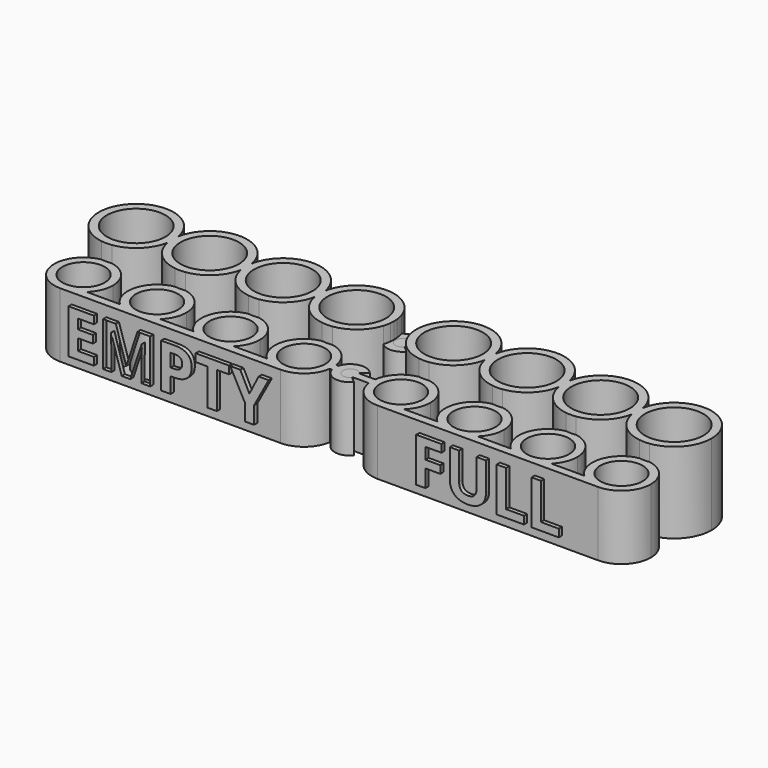
from build123d import *

# Parameters (mm, degrees)
F0_R         = 7.25
F1_DEPTH     = 20
F0_R_2       = 5.25
F2_DEPTH     = 16
F3_DEPTH     = 1.6
F4_TEXT_SIZE = 15.2777777778
F5_DEPTH     = 1
F6_DEPTH     = 20
F7_DEPTH     = 16
F8_TEXT_SIZE = 15.2777777778
F9_DEPTH     = 1
F10_DEPTH    = 1.6


# Not quite as in the source:
# - a feature names something its author has since deleted; it is built from what else it names
# - Text() gives the source's letters only with a copy of the font that has no kerning and outlines rounded to 1/6400 em; it was checked with that copy


with BuildPart() as f1:
    # F0 (on Top) → F1 (new body)
    with BuildSketch(Plane.XY):
        with BuildLine():
            ThreePointArc((-15.1805921053, -2.7893627205), (-16.4, 0), (-15.1805921053, 2.7893627205))
            ThreePointArc((-15.1805921053, 2.7893627205), (-24.5823020266, 9.231653392), (-33.1, 1.6590660023))
            ThreePointArc((-33.1, 1.6590660023), (-32.9875763232, 0.8329165624), (-32.95, 0))
            ThreePointArc((-32.95, 0), (-32.9875763232, -0.8329165624), (-33.1, -1.6590660023))
            ThreePointArc((-33.1, -1.6590660023), (-30.4002858895, -6.678236334), (-25.2709482961, -9.1622699387))
            ThreePointArc((-25.2709482961, -9.1622699387), (-24, -9.05), (-22.7290517039, -9.1622699387))
            ThreePointArc((-22.7290517039, -9.1622699387), (-18.0328140118, -7.067898654), (-15.1805921053, -2.7893627205))
        make_face()
        with Locations((-24, 0)):
            Circle(F0_R, mode=Mode.SUBTRACT)
        with BuildLine():
            ThreePointArc((-14.8042129211, 1), (-14.9480793629, 1.9040044063), (-15.1805921053, 2.7893627205))
            ThreePointArc((-15.1805921053, 2.7893627205), (-16.4, 0), (-15.1805921053, -2.7893627205))
            ThreePointArc((-15.1805921053, -2.7893627205), (-14.9480793629, -1.9040044063), (-14.8042129211, -1))
            ThreePointArc((-14.8042129211, -1), (-14.763563174, -0.5007342211), (-14.75, 0))
            ThreePointArc((-14.75, 0), (-14.763563174, 0.5007342211), (-14.8042129211, 1))
        make_face()
        with BuildLine():
            ThreePointArc((-32.95, 0), (-32.9875763232, 0.8329165624), (-33.1, 1.6590660023))
            ThreePointArc((-33.1, 1.6590660023), (-33.25, 0), (-33.1, -1.6590660023))
            ThreePointArc((-33.1, -1.6590660023), (-32.9875763232, -0.8329165624), (-32.95, 0))
        make_face()
        with BuildLine():
            ThreePointArc((-33.1, -1.6590660023), (-33.25, 0), (-33.1, 1.6590660023))
            ThreePointArc((-33.1, 1.6590660023), (-42.2, 9.25), (-51.3, 1.6590660023))
            ThreePointArc((-51.3, 1.6590660023), (-51.1875763232, 0.8329165624), (-51.15, 0))
            ThreePointArc((-51.15, 0), (-51.1875763232, -0.8329165624), (-51.3, -1.6590660023))
            ThreePointArc((-51.3, -1.6590660023), (-48.6002858895, -6.678236334), (-43.4709482961, -9.1622699387))
            ThreePointArc((-43.4709482961, -9.1622699387), (-42.2, -9.05), (-40.9290517039, -9.1622699387))
            ThreePointArc((-40.9290517039, -9.1622699387), (-35.7997141105, -6.678236334), (-33.1, -1.6590660023))
        make_face()
        with Locations((-42.2, 0)):
            Circle(F0_R, mode=Mode.SUBTRACT)
        with BuildLine():
            ThreePointArc((-25.2709482961, -9.1622699387), (-24, -9.25), (-22.7290517039, -9.1622699387))
            ThreePointArc((-22.7290517039, -9.1622699387), (-24, -9.05), (-25.2709482961, -9.1622699387))
        make_face()
        with BuildLine():
            ThreePointArc((-51.15, 0), (-51.1875763232, 0.8329165624), (-51.3, 1.6590660023))
            ThreePointArc((-51.3, 1.6590660023), (-51.45, 0), (-51.3, -1.6590660023))
            ThreePointArc((-51.3, -1.6590660023), (-51.1875763232, -0.8329165624), (-51.15, 0))
        make_face()
        with BuildLine():
            ThreePointArc((-51.3, -1.6590660023), (-51.45, 0), (-51.3, 1.6590660023))
            ThreePointArc((-51.3, 1.6590660023), (-60.4, 9.25), (-69.5, 1.6590660023))
            ThreePointArc((-69.5, 1.6590660023), (-69.3875763232, 0.8329165624), (-69.35, 0))
            ThreePointArc((-69.35, 0), (-69.3875763232, -0.8329165624), (-69.5, -1.6590660023))
            ThreePointArc((-69.5, -1.6590660023), (-66.8002858895, -6.678236334), (-61.6709482961, -9.1622699387))
            ThreePointArc((-61.6709482961, -9.1622699387), (-60.4, -9.05), (-59.1290517039, -9.1622699387))
            ThreePointArc((-59.1290517039, -9.1622699387), (-53.9997141105, -6.678236334), (-51.3, -1.6590660023))
        make_face()
        with Locations((-60.4, 0)):
            Circle(F0_R, mode=Mode.SUBTRACT)
        with BuildLine():
            ThreePointArc((-43.4709482961, -9.1622699387), (-42.2, -9.25), (-40.9290517039, -9.1622699387))
            ThreePointArc((-40.9290517039, -9.1622699387), (-42.2, -9.05), (-43.4709482961, -9.1622699387))
        make_face()
        with BuildLine():
            ThreePointArc((-69.35, 0), (-69.3875763232, 0.8329165624), (-69.5, 1.6590660023))
            ThreePointArc((-69.5, 1.6590660023), (-69.65, 0), (-69.5, -1.6590660023))
            ThreePointArc((-69.5, -1.6590660023), (-69.3875763232, -0.8329165624), (-69.35, 0))
        make_face()
        with BuildLine():
            ThreePointArc((-69.5, -1.6590660023), (-69.65, 0), (-69.5, 1.6590660023))
            ThreePointArc((-69.5, 1.6590660023), (-85.278236334, 6.4002858895), (-79.8709482961, -9.1622699387))
            ThreePointArc((-79.8709482961, -9.1622699387), (-78.6, -9.05), (-77.3290517039, -9.1622699387))
            ThreePointArc((-77.3290517039, -9.1622699387), (-72.1997141105, -6.678236334), (-69.5, -1.6590660023))
        make_face()
        with Locations((-78.6, 0)):
            Circle(F0_R, mode=Mode.SUBTRACT)
        with BuildLine():
            ThreePointArc((-61.6709482961, -9.1622699387), (-60.4, -9.25), (-59.1290517039, -9.1622699387))
            ThreePointArc((-59.1290517039, -9.1622699387), (-60.4, -9.05), (-61.6709482961, -9.1622699387))
        make_face()
        with BuildLine():
            ThreePointArc((-77.3290517039, -9.1622699387), (-78.6, -9.05), (-79.8709482961, -9.1622699387))
            ThreePointArc((-79.8709482961, -9.1622699387), (-78.6, -9.25), (-77.3290517039, -9.1622699387))
        make_face()
    extrude(amount=F1_DEPTH)

    # F0 (on Top) → F2 (join)
    with BuildSketch(Plane.XY):
        with BuildLine():
            Line((-16.266060556, -15.3), (-16.8192966918, -15.3))
            ThreePointArc((-16.8192966918, -15.3), (-16.767344921, -15.7988009299), (-16.75, -16.3))
            ThreePointArc((-16.75, -16.3), (-16.767344921, -16.8011990701), (-16.8192966918, -17.3))
            Line((-16.8192966918, -17.3), (-16.266060556, -17.3))
            ThreePointArc((-16.266060556, -17.3), (-16.4, -16.3), (-16.266060556, -15.3))
        make_face()
        with BuildLine():
            Line((-14.0966629547, -15.3), (-16.266060556, -15.3))
            ThreePointArc((-16.266060556, -15.3), (-16.4, -16.3), (-16.266060556, -17.3))
            Line((-16.266060556, -17.3), (-14.0966629547, -17.3))
            ThreePointArc((-14.0966629547, -17.3), (-14.4, -16.3), (-14.0966629547, -15.3))
        make_face()
        with BuildLine():
            ThreePointArc((-77.3290517039, -9.1622699387), (-78.6, -9.25), (-79.8709482961, -9.1622699387))
            ThreePointArc((-79.8709482961, -9.1622699387), (-85.8218779741, -16.9379486873), (-78.6, -23.55))
            ThreePointArc((-78.6, -23.55), (-75.9074175964, -23.0314560089), (-73.6, -21.55))
            ThreePointArc((-73.6, -21.55), (-71.9361985324, -19.1559149147), (-71.35, -16.3))
            ThreePointArc((-71.35, -16.3), (-73.0422632688, -11.6444589545), (-77.3290517039, -9.1622699387))
        make_face()
        with Locations((-78.6, -16.3)):
            Circle(F0_R_2, mode=Mode.SUBTRACT)
        with BuildLine():
            ThreePointArc((-73.6, -21.55), (-75.9074175964, -23.0314560089), (-78.6, -23.55))
            Line((-78.6, -23.55), (-60.4, -23.55))
            ThreePointArc((-60.4, -23.55), (-63.0925824036, -23.0314560089), (-65.4, -21.55))
            Line((-65.4, -21.55), (-73.6, -21.55))
        make_face()
        with BuildLine():
            ThreePointArc((-53.15, -16.3), (-54.8422632688, -11.6444589545), (-59.1290517039, -9.1622699387))
            ThreePointArc((-59.1290517039, -9.1622699387), (-60.4, -9.25), (-61.6709482961, -9.1622699387))
            ThreePointArc((-61.6709482961, -9.1622699387), (-67.3422735578, -14.2101823408), (-65.4, -21.55))
            ThreePointArc((-65.4, -21.55), (-63.0925824036, -23.0314560089), (-60.4, -23.55))
            ThreePointArc((-60.4, -23.55), (-57.7074175964, -23.0314560089), (-55.4, -21.55))
            ThreePointArc((-55.4, -21.55), (-53.7361985324, -19.1559149147), (-53.15, -16.3))
        make_face()
        with Locations((-60.4, -16.3)):
            Circle(F0_R_2, mode=Mode.SUBTRACT)
        with BuildLine():
            ThreePointArc((-42.2, -23.55), (-44.8925824036, -23.0314560089), (-47.2, -21.55))
            Line((-47.2, -21.55), (-55.4, -21.55))
            ThreePointArc((-55.4, -21.55), (-57.7074175964, -23.0314560089), (-60.4, -23.55))
            Line((-60.4, -23.55), (-42.2, -23.55))
        make_face()
        with BuildLine():
            ThreePointArc((-34.95, -16.3), (-36.6422632688, -11.6444589545), (-40.9290517039, -9.1622699387))
            ThreePointArc((-40.9290517039, -9.1622699387), (-42.2, -9.25), (-43.4709482961, -9.1622699387))
            ThreePointArc((-43.4709482961, -9.1622699387), (-49.1422735578, -14.2101823408), (-47.2, -21.55))
            ThreePointArc((-47.2, -21.55), (-44.8925824036, -23.0314560089), (-42.2, -23.55))
            ThreePointArc((-42.2, -23.55), (-39.5074175964, -23.0314560089), (-37.2, -21.55))
            ThreePointArc((-37.2, -21.55), (-35.5361985324, -19.1559149147), (-34.95, -16.3))
        make_face()
        with Locations((-42.2, -16.3)):
            Circle(F0_R_2, mode=Mode.SUBTRACT)
        with BuildLine():
            ThreePointArc((-24, -23.55), (-26.6925824036, -23.0314560089), (-29, -21.55))
            Line((-29, -21.55), (-37.2, -21.55))
            ThreePointArc((-37.2, -21.55), (-39.5074175964, -23.0314560089), (-42.2, -23.55))
            Line((-42.2, -23.55), (-24, -23.55))
        make_face()
        with BuildLine():
            ThreePointArc((-16.8192966918, -15.3), (-18.7774013857, -11.2713855076), (-22.7290517039, -9.1622699387))
            ThreePointArc((-22.7290517039, -9.1622699387), (-24, -9.25), (-25.2709482961, -9.1622699387))
            ThreePointArc((-25.2709482961, -9.1622699387), (-30.9422735578, -14.2101823408), (-29, -21.55))
            ThreePointArc((-29, -21.55), (-26.6925824036, -23.0314560089), (-24, -23.55))
            ThreePointArc((-24, -23.55), (-19.2401418088, -21.7686607136), (-16.8192966918, -17.3))
            ThreePointArc((-16.8192966918, -17.3), (-16.767344921, -16.8011990701), (-16.75, -16.3))
            ThreePointArc((-16.75, -16.3), (-16.767344921, -15.7988009299), (-16.8192966918, -15.3))
        make_face()
        with Locations((-24, -16.3)):
            Circle(F0_R_2, mode=Mode.SUBTRACT)
        with BuildLine():
            Line((-11.2211200024, 1.1570176974), (-9.6890311161, 2.4425929168))
            ThreePointArc((-9.6890311161, 2.4425929168), (-12.3605223849, 3.7924465022), (-15.1805921053, 2.7893627205))
            ThreePointArc((-15.1805921053, 2.7893627205), (-14.9480793629, 1.9040044063), (-14.8042129211, 1))
            Line((-14.8042129211, 1), (-14.0966629547, 1))
            ThreePointArc((-14.0966629547, 1), (-12.6981419664, 1.7973224959), (-11.2211200024, 1.1570176974))
        make_face()
        with BuildLine():
            ThreePointArc((-14.0966629547, -1), (-14.4, 0), (-14.0966629547, 1))
            Line((-14.0966629547, 1), (-14.8042129211, 1))
            ThreePointArc((-14.8042129211, 1), (-14.763563174, 0.5007342211), (-14.75, 0))
            ThreePointArc((-14.75, 0), (-14.763563174, -0.5007342211), (-14.8042129211, -1))
            Line((-14.8042129211, -1), (-14.0966629547, -1))
        make_face()
        with BuildLine():
            ThreePointArc((-15.1805921053, -2.7893627205), (-12.3605223849, -3.7924465022), (-9.6890311161, -2.4425929168))
            Line((-9.6890311161, -2.4425929168), (-11.2211200024, -1.1570176974))
            ThreePointArc((-11.2211200024, -1.1570176974), (-12.6981419664, -1.7973224959), (-14.0966629547, -1))
            Line((-14.0966629547, -1), (-14.8042129211, -1))
            ThreePointArc((-14.8042129211, -1), (-14.9480793629, -1.9040044063), (-15.1805921053, -2.7893627205))
        make_face()
        with BuildLine():
            Line((-11.2211200024, -15.1429823026), (-9.6890311161, -13.8574070832))
            ThreePointArc((-9.6890311161, -13.8574070832), (-13.4141310946, -12.5882361928), (-16.266060556, -15.3))
            Line((-16.266060556, -15.3), (-14.0966629547, -15.3))
            ThreePointArc((-14.0966629547, -15.3), (-12.6981419664, -14.5026775041), (-11.2211200024, -15.1429823026))
        make_face()
        with BuildLine():
            ThreePointArc((-16.266060556, -17.3), (-13.4141310946, -20.0117638072), (-9.6890311161, -18.7425929168))
            Line((-9.6890311161, -18.7425929168), (-11.2211200024, -17.4570176974))
            ThreePointArc((-11.2211200024, -17.4570176974), (-12.6981419664, -18.0973224959), (-14.0966629547, -17.3))
            Line((-14.0966629547, -17.3), (-16.266060556, -17.3))
        make_face()
    extrude(amount=F2_DEPTH)

    # F0 (on Top) → F3 (join)
    with BuildSketch(Plane.XY):
        with Locations((-42.2, 0)):
            Circle(F0_R)
        with Locations((-24, 0)):
            Circle(F0_R)
        with Locations((-60.4, 0)):
            Circle(F0_R)
        with Locations((-78.6, 0)):
            Circle(F0_R)
        with Locations((-24, -16.3)):
            Circle(F0_R_2)
        with Locations((-42.2, -16.3)):
            Circle(F0_R_2)
        with Locations((-60.4, -16.3)):
            Circle(F0_R_2)
        with Locations((-78.6, -16.3)):
            Circle(F0_R_2)
    extrude(amount=F3_DEPTH)

    # F4 (on face) → F5 (join)
    with BuildSketch(Plane.XZ.offset(23.55)):
        with Locations((-77.1, 2.5)):
            Text('EMPTY', F4_TEXT_SIZE, font='Open Sans', font_style=FontStyle.BOLD, text_align=(TextAlign.LEFT, TextAlign.BOTTOM))
    extrude(amount=F5_DEPTH)


with BuildPart() as f6:
    # F0 (on Top) → F6 (new body)
    with BuildSketch(Plane.XY):
        with BuildLine():
            ThreePointArc((9.1, 1.6590660023), (-0.0647103616, 9.2497736496), (-9.1223214286, 1.5315847198))
            ThreePointArc((-9.1223214286, 1.5315847198), (-8.8814533369, 0.7825667475), (-8.8, 0))
            ThreePointArc((-8.8, 0), (-8.8814533369, -0.7825667475), (-9.1223214286, -1.5315847198))
            ThreePointArc((-9.1223214286, -1.5315847198), (-6.446848309, -6.633298341), (-1.2709482961, -9.1622699387))
            ThreePointArc((-1.2709482961, -9.1622699387), (0, -9.05), (1.2709482961, -9.1622699387))
            ThreePointArc((1.2709482961, -9.1622699387), (6.4002858895, -6.678236334), (9.1, -1.6590660023))
            ThreePointArc((9.1, -1.6590660023), (8.95, 0), (9.1, 1.6590660023))
        make_face()
        Circle(F0_R, mode=Mode.SUBTRACT)
        with BuildLine():
            ThreePointArc((-9.1223214286, 1.5315847198), (-9.16291004, 1.2663252342), (-9.1957870789, 1))
            ThreePointArc((-9.1957870789, 1), (-9.25, 0), (-9.1957870789, -1))
            ThreePointArc((-9.1957870789, -1), (-9.16291004, -1.2663252342), (-9.1223214286, -1.5315847198))
            ThreePointArc((-9.1223214286, -1.5315847198), (-8.8814533369, -0.7825667475), (-8.8, 0))
            ThreePointArc((-8.8, 0), (-8.8814533369, 0.7825667475), (-9.1223214286, 1.5315847198))
        make_face()
        with BuildLine():
            ThreePointArc((9.25, 0), (9.2124236768, 0.8329165624), (9.1, 1.6590660023))
            ThreePointArc((9.1, 1.6590660023), (8.95, 0), (9.1, -1.6590660023))
            ThreePointArc((9.1, -1.6590660023), (9.2124236768, -0.8329165624), (9.25, 0))
        make_face()
        with BuildLine():
            ThreePointArc((27.3, 1.6590660023), (18.2, 9.25), (9.1, 1.6590660023))
            ThreePointArc((9.1, 1.6590660023), (9.2124236768, 0.8329165624), (9.25, 0))
            ThreePointArc((9.25, 0), (9.2124236768, -0.8329165624), (9.1, -1.6590660023))
            ThreePointArc((9.1, -1.6590660023), (11.7997141105, -6.678236334), (16.9290517039, -9.1622699387))
            ThreePointArc((16.9290517039, -9.1622699387), (18.2, -9.05), (19.4709482961, -9.1622699387))
            ThreePointArc((19.4709482961, -9.1622699387), (24.6002858895, -6.678236334), (27.3, -1.6590660023))
            ThreePointArc((27.3, -1.6590660023), (27.15, 0), (27.3, 1.6590660023))
        make_face()
        with Locations((18.2, 0)):
            Circle(F0_R, mode=Mode.SUBTRACT)
        with BuildLine():
            ThreePointArc((27.45, 0), (27.4124236768, 0.8329165624), (27.3, 1.6590660023))
            ThreePointArc((27.3, 1.6590660023), (27.15, 0), (27.3, -1.6590660023))
            ThreePointArc((27.3, -1.6590660023), (27.4124236768, -0.8329165624), (27.45, 0))
        make_face()
        with BuildLine():
            ThreePointArc((45.5, 1.6590660023), (36.4, 9.25), (27.3, 1.6590660023))
            ThreePointArc((27.3, 1.6590660023), (27.4124236768, 0.8329165624), (27.45, 0))
            ThreePointArc((27.45, 0), (27.4124236768, -0.8329165624), (27.3, -1.6590660023))
            ThreePointArc((27.3, -1.6590660023), (29.9997141105, -6.678236334), (35.1290517039, -9.1622699387))
            ThreePointArc((35.1290517039, -9.1622699387), (36.4, -9.05), (37.6709482961, -9.1622699387))
            ThreePointArc((37.6709482961, -9.1622699387), (42.8002858895, -6.678236334), (45.5, -1.6590660023))
            ThreePointArc((45.5, -1.6590660023), (45.35, 0), (45.5, 1.6590660023))
        make_face()
        with Locations((36.4, 0)):
            Circle(F0_R, mode=Mode.SUBTRACT)
        with BuildLine():
            ThreePointArc((45.65, 0), (45.6124236768, 0.8329165624), (45.5, 1.6590660023))
            ThreePointArc((45.5, 1.6590660023), (45.35, 0), (45.5, -1.6590660023))
            ThreePointArc((45.5, -1.6590660023), (45.6124236768, -0.8329165624), (45.65, 0))
        make_face()
        with BuildLine():
            ThreePointArc((63.85, 0), (55.4329165624, 9.2124236768), (45.5, 1.6590660023))
            ThreePointArc((45.5, 1.6590660023), (45.6124236768, 0.8329165624), (45.65, 0))
            ThreePointArc((45.65, 0), (45.6124236768, -0.8329165624), (45.5, -1.6590660023))
            ThreePointArc((45.5, -1.6590660023), (48.1997141105, -6.678236334), (53.3290517039, -9.1622699387))
            ThreePointArc((53.3290517039, -9.1622699387), (54.6, -9.05), (55.8709482961, -9.1622699387))
            ThreePointArc((55.8709482961, -9.1622699387), (61.575627991, -6.0747933406), (63.85, 0))
        make_face()
        with Locations((54.6, 0)):
            Circle(F0_R, mode=Mode.SUBTRACT)
        with BuildLine():
            ThreePointArc((1.2709482961, -9.1622699387), (0, -9.05), (-1.2709482961, -9.1622699387))
            ThreePointArc((-1.2709482961, -9.1622699387), (0, -9.25), (1.2709482961, -9.1622699387))
        make_face()
        with BuildLine():
            ThreePointArc((19.4709482961, -9.1622699387), (18.2, -9.05), (16.9290517039, -9.1622699387))
            ThreePointArc((16.9290517039, -9.1622699387), (18.2, -9.25), (19.4709482961, -9.1622699387))
        make_face()
        with BuildLine():
            ThreePointArc((37.6709482961, -9.1622699387), (36.4, -9.05), (35.1290517039, -9.1622699387))
            ThreePointArc((35.1290517039, -9.1622699387), (36.4, -9.25), (37.6709482961, -9.1622699387))
        make_face()
        with BuildLine():
            ThreePointArc((53.3290517039, -9.1622699387), (54.6, -9.25), (55.8709482961, -9.1622699387))
            ThreePointArc((55.8709482961, -9.1622699387), (54.6, -9.05), (53.3290517039, -9.1622699387))
        make_face()
    extrude(amount=F6_DEPTH)

    # F0 (on Top) → F7 (join)
    with BuildSketch(Plane.XY):
        with BuildLine():
            Line((-14.0966629547, 1), (-11.4082464074, 1))
            Line((-11.4082464074, 1), (-11.2211200024, 1.1570176974))
            ThreePointArc((-11.2211200024, 1.1570176974), (-12.6981419664, 1.7973224959), (-14.0966629547, 1))
        make_face()
        with BuildLine():
            Line((-12.6, 0), (-11.4082464074, 1))
            Line((-11.4082464074, 1), (-14.0966629547, 1))
            ThreePointArc((-14.0966629547, 1), (-14.4, 0), (-14.0966629547, -1))
            Line((-14.0966629547, -1), (-11.4082464074, -1))
            Line((-11.4082464074, -1), (-12.6, 0))
        make_face()
        with BuildLine():
            Line((-11.2211200024, -1.1570176974), (-11.4082464074, -1))
            Line((-11.4082464074, -1), (-14.0966629547, -1))
            ThreePointArc((-14.0966629547, -1), (-12.6981419664, -1.7973224959), (-11.2211200024, -1.1570176974))
        make_face()
        with BuildLine():
            ThreePointArc((-10.8, 0), (-10.877502784, 0.522497216), (-11.1033370453, 1))
            Line((-11.1033370453, 1), (-11.4082464074, 1))
            Line((-11.4082464074, 1), (-12.6, 0))
            Line((-12.6, 0), (-11.4082464074, -1))
            Line((-11.4082464074, -1), (-11.1033370453, -1))
            ThreePointArc((-11.1033370453, -1), (-10.877502784, -0.522497216), (-10.8, 0))
        make_face()
        with BuildLine():
            Line((-11.4082464074, 1), (-11.1033370453, 1))
            ThreePointArc((-11.1033370453, 1), (-11.1600866495, 1.080115523), (-11.2211200024, 1.1570176974))
            Line((-11.2211200024, 1.1570176974), (-11.4082464074, 1))
        make_face()
        with BuildLine():
            ThreePointArc((-11.2211200024, -1.1570176974), (-11.1600866495, -1.080115523), (-11.1033370453, -1))
            Line((-11.1033370453, -1), (-11.4082464074, -1))
            Line((-11.4082464074, -1), (-11.2211200024, -1.1570176974))
        make_face()
        with BuildLine():
            ThreePointArc((-9.1957870789, -1), (-9.25, 0), (-9.1957870789, 1))
            Line((-9.1957870789, 1), (-11.1033370453, 1))
            ThreePointArc((-11.1033370453, 1), (-10.877502784, 0.522497216), (-10.8, 0))
            ThreePointArc((-10.8, 0), (-10.877502784, -0.522497216), (-11.1033370453, -1))
            Line((-11.1033370453, -1), (-9.1957870789, -1))
        make_face()
        with BuildLine():
            Line((-14.0966629547, -15.3), (-11.4082464074, -15.3))
            Line((-11.4082464074, -15.3), (-11.2211200024, -15.1429823026))
            ThreePointArc((-11.2211200024, -15.1429823026), (-12.6981419664, -14.5026775041), (-14.0966629547, -15.3))
        make_face()
        with BuildLine():
            Line((-12.6, -16.3), (-11.4082464074, -15.3))
            Line((-11.4082464074, -15.3), (-14.0966629547, -15.3))
            ThreePointArc((-14.0966629547, -15.3), (-14.4, -16.3), (-14.0966629547, -17.3))
            Line((-14.0966629547, -17.3), (-11.4082464074, -17.3))
            Line((-11.4082464074, -17.3), (-12.6, -16.3))
        make_face()
        with BuildLine():
            Line((-11.2211200024, -17.4570176974), (-11.4082464074, -17.3))
            Line((-11.4082464074, -17.3), (-14.0966629547, -17.3))
            ThreePointArc((-14.0966629547, -17.3), (-12.6981419664, -18.0973224959), (-11.2211200024, -17.4570176974))
        make_face()
        with BuildLine():
            ThreePointArc((-11.2211200024, -17.4570176974), (-11.1600866495, -17.380115523), (-11.1033370453, -17.3))
            Line((-11.1033370453, -17.3), (-11.4082464074, -17.3))
            Line((-11.4082464074, -17.3), (-11.2211200024, -17.4570176974))
        make_face()
        with BuildLine():
            ThreePointArc((-10.8, -16.3), (-10.877502784, -15.777502784), (-11.1033370453, -15.3))
            Line((-11.1033370453, -15.3), (-11.4082464074, -15.3))
            Line((-11.4082464074, -15.3), (-12.6, -16.3))
            Line((-12.6, -16.3), (-11.4082464074, -17.3))
            Line((-11.4082464074, -17.3), (-11.1033370453, -17.3))
            ThreePointArc((-11.1033370453, -17.3), (-10.877502784, -16.822497216), (-10.8, -16.3))
        make_face()
        with BuildLine():
            Line((-11.4082464074, -15.3), (-11.1033370453, -15.3))
            ThreePointArc((-11.1033370453, -15.3), (-11.1600866495, -15.219884477), (-11.2211200024, -15.1429823026))
            Line((-11.2211200024, -15.1429823026), (-11.4082464074, -15.3))
        make_face()
        with BuildLine():
            ThreePointArc((-8.8, -16.3), (-8.8336337066, -15.7955349926), (-8.933939444, -15.3))
            Line((-8.933939444, -15.3), (-11.1033370453, -15.3))
            ThreePointArc((-11.1033370453, -15.3), (-10.877502784, -15.777502784), (-10.8, -16.3))
            ThreePointArc((-10.8, -16.3), (-10.877502784, -16.822497216), (-11.1033370453, -17.3))
            Line((-11.1033370453, -17.3), (-8.933939444, -17.3))
            ThreePointArc((-8.933939444, -17.3), (-8.8336337066, -16.8044650074), (-8.8, -16.3))
        make_face()
        with BuildLine():
            ThreePointArc((-7.1807033082, -17.3), (-7.25, -16.3), (-7.1807033082, -15.3))
            Line((-7.1807033082, -15.3), (-8.933939444, -15.3))
            ThreePointArc((-8.933939444, -15.3), (-8.8336337066, -15.7955349926), (-8.8, -16.3))
            ThreePointArc((-8.8, -16.3), (-8.8336337066, -16.8044650074), (-8.933939444, -17.3))
            Line((-8.933939444, -17.3), (-7.1807033082, -17.3))
        make_face()
        with BuildLine():
            ThreePointArc((1.2709482961, -9.1622699387), (0, -9.25), (-1.2709482961, -9.1622699387))
            ThreePointArc((-1.2709482961, -9.1622699387), (-5.2225986143, -11.2713855076), (-7.1807033082, -15.3))
            ThreePointArc((-7.1807033082, -15.3), (-7.25, -16.3), (-7.1807033082, -17.3))
            ThreePointArc((-7.1807033082, -17.3), (-4.7598581912, -21.7686607136), (0, -23.55))
            ThreePointArc((0, -23.55), (2.6925824036, -23.0314560089), (5, -21.55))
            ThreePointArc((5, -21.55), (6.6638014676, -19.1559149147), (7.25, -16.3))
            ThreePointArc((7.25, -16.3), (5.5577367312, -11.6444589545), (1.2709482961, -9.1622699387))
        make_face()
        with Locations((0, -16.3)):
            Circle(F0_R_2, mode=Mode.SUBTRACT)
        with BuildLine():
            ThreePointArc((18.2, -23.55), (15.5074175964, -23.0314560089), (13.2, -21.55))
            Line((13.2, -21.55), (5, -21.55))
            ThreePointArc((5, -21.55), (2.6925824036, -23.0314560089), (0, -23.55))
            Line((0, -23.55), (18.2, -23.55))
        make_face()
        with BuildLine():
            ThreePointArc((19.4709482961, -9.1622699387), (18.2, -9.25), (16.9290517039, -9.1622699387))
            ThreePointArc((16.9290517039, -9.1622699387), (11.2577264422, -14.2101823408), (13.2, -21.55))
            ThreePointArc((13.2, -21.55), (15.5074175964, -23.0314560089), (18.2, -23.55))
            ThreePointArc((18.2, -23.55), (20.8925824036, -23.0314560089), (23.2, -21.55))
            ThreePointArc((23.2, -21.55), (24.8638014676, -19.1559149147), (25.45, -16.3))
            ThreePointArc((25.45, -16.3), (23.7577367312, -11.6444589545), (19.4709482961, -9.1622699387))
        make_face()
        with Locations((18.2, -16.3)):
            Circle(F0_R_2, mode=Mode.SUBTRACT)
        with BuildLine():
            ThreePointArc((36.4, -23.55), (33.7074175964, -23.0314560089), (31.4, -21.55))
            Line((31.4, -21.55), (23.2, -21.55))
            ThreePointArc((23.2, -21.55), (20.8925824036, -23.0314560089), (18.2, -23.55))
            Line((18.2, -23.55), (36.4, -23.55))
        make_face()
        with BuildLine():
            ThreePointArc((37.6709482961, -9.1622699387), (36.4, -9.25), (35.1290517039, -9.1622699387))
            ThreePointArc((35.1290517039, -9.1622699387), (29.4577264422, -14.2101823408), (31.4, -21.55))
            ThreePointArc((31.4, -21.55), (33.7074175964, -23.0314560089), (36.4, -23.55))
            ThreePointArc((36.4, -23.55), (39.0925824036, -23.0314560089), (41.4, -21.55))
            ThreePointArc((41.4, -21.55), (43.0638014676, -19.1559149147), (43.65, -16.3))
            ThreePointArc((43.65, -16.3), (41.9577367312, -11.6444589545), (37.6709482961, -9.1622699387))
        make_face()
        with Locations((36.4, -16.3)):
            Circle(F0_R_2, mode=Mode.SUBTRACT)
        with BuildLine():
            ThreePointArc((54.6, -23.55), (51.9074175964, -23.0314560089), (49.6, -21.55))
            Line((49.6, -21.55), (41.4, -21.55))
            ThreePointArc((41.4, -21.55), (39.0925824036, -23.0314560089), (36.4, -23.55))
            Line((36.4, -23.55), (54.6, -23.55))
        make_face()
        with BuildLine():
            ThreePointArc((61.85, -16.3), (60.1577367312, -11.6444589545), (55.8709482961, -9.1622699387))
            ThreePointArc((55.8709482961, -9.1622699387), (54.6, -9.25), (53.3290517039, -9.1622699387))
            ThreePointArc((53.3290517039, -9.1622699387), (47.6577264422, -14.2101823408), (49.6, -21.55))
            ThreePointArc((49.6, -21.55), (51.9074175964, -23.0314560089), (54.6, -23.55))
            ThreePointArc((54.6, -23.55), (59.7265241636, -21.4265241636), (61.85, -16.3))
        make_face()
        with Locations((54.6, -16.3)):
            Circle(F0_R_2, mode=Mode.SUBTRACT)
    extrude(amount=F7_DEPTH)

    # F8 (on face) → F9 (join)
    with BuildSketch(Plane.XZ.offset(23.55)):
        with Locations((9, 2.5)):
            Text('FULL', F8_TEXT_SIZE, font='Open Sans', font_style=FontStyle.BOLD, text_align=(TextAlign.LEFT, TextAlign.BOTTOM))
    extrude(amount=F9_DEPTH)

    # F0 (on Top) → F10 (join)
    with BuildSketch(Plane.XY):
        Circle(F0_R)
        with Locations((18.2, 0)):
            Circle(F0_R)
        with Locations((36.4, 0)):
            Circle(F0_R)
        with Locations((54.6, 0)):
            Circle(F0_R)
        with Locations((54.6, -16.3)):
            Circle(F0_R_2)
        with Locations((36.4, -16.3)):
            Circle(F0_R_2)
        with Locations((18.2, -16.3)):
            Circle(F0_R_2)
        with Locations((0, -16.3)):
            Circle(F0_R_2)
    extrude(amount=F10_DEPTH)


solid = Compound([f1.part, f6.part])
